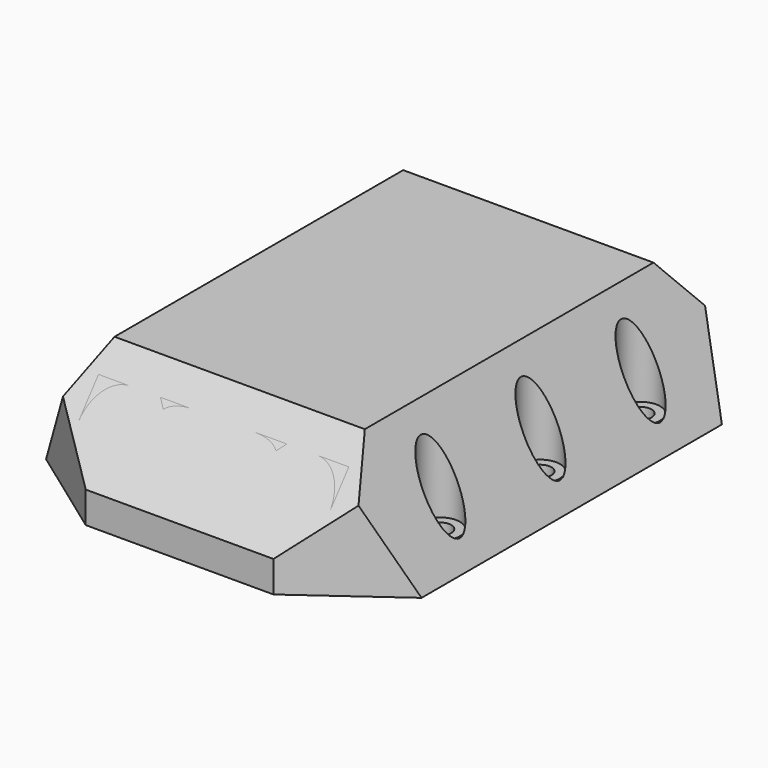
from build123d import *

# Parameters (mm, degrees)
F0_R         = 3.125
F1_DEPTH     = 20
F2_START     = 16
F2_DEPTH     = 4
F3_T1_DEPTH  = 163.5931549515
F4_SIZE2     = 15
F4_SIZE      = 12
F0_R_2       = 1.75
F5_DEPTH     = 4
F6_SIZE2     = 15
F6_SIZE      = 5
F7_T1_DEPTH  = 38.5354006484
F7_T6_DEPTH  = 25.1531696001
F7_T12_DEPTH = 74.7709385518
F7_T18_DEPTH = 25.1531696001
F7_T24_DEPTH = 25.1531696001
F7_T30_DEPTH = 74.7709385518
F7_T36_DEPTH = 25.1531696001


# Not quite as in the source:
# - a fillet or chamfer that OpenCascade refuses, or shapes differently, is made with other operations: its cross-section is extruded or revolved along the edge and cut away or added


with BuildPart() as f1:
    # F0 (on Top) → F1 (new body)
    with BuildSketch(Plane.XY):
        Polygon((-15, 40.8282039139), (-30, 30), (-30, -30), (-15, -40.8282039139), (15, -40.8282039139), (30, -30), (30, 30), (15, 40.8282039139), align=None)
        with Locations((-25, -20)):
            Circle(F0_R, mode=Mode.SUBTRACT)
        with Locations((25, -20)):
            Circle(F0_R, mode=Mode.SUBTRACT)
        with Locations((-25, 0)):
            Circle(F0_R, mode=Mode.SUBTRACT)
        with Locations((-25, 20)):
            Circle(F0_R, mode=Mode.SUBTRACT)
        Polygon((-11.7677003242, -30.8282039139), (-20, -24.8854692759), (-20, 24.8854692759), (-11.7677003242, 30.8282039139), (11.7677003242, 30.8282039139), (20, 24.8854692759), (20, -24.8854692759), (11.7677003242, -30.8282039139), align=None, mode=Mode.SUBTRACT)
        with Locations((25, 0)):
            Circle(F0_R, mode=Mode.SUBTRACT)
        with Locations((25, 20)):
            Circle(F0_R, mode=Mode.SUBTRACT)
    extrude(amount=F1_DEPTH)

    # F0 (on Top) → F2 (join)
    with BuildSketch(Plane.XY.offset(F2_START)):
        Polygon((-20, 24.8854692759), (-20, -24.8854692759), (-11.7677003242, -30.8282039139), (11.7677003242, -30.8282039139), (20, -24.8854692759), (20, 24.8854692759), (11.7677003242, 30.8282039139), (-11.7677003242, 30.8282039139), align=None)
    extrude(amount=F2_DEPTH)

    # F3: chamfer of 10 x 20 on 2 edges, made by hand

    # F3_s2 → F3_t1 (cut)
    with BuildSketch(Plane.XZ.offset(-81.7965774757)):
        Polygon((-30, 0), (-20, 20), (-30, 20), align=None)
        Polygon((20, 20), (30, 0), (30, 20), align=None)
    extrude(amount=F3_T1_DEPTH, mode=Mode.SUBTRACT)

    # F4
    f4_edges = [f1.edges().sort_by_distance(p)[0] for p in [
        (0, -40.828204, 20),
        (0, 40.828204, 20),
    ]]
    f4_side = f1.faces().sort_by_distance((0, 0, 20))[0]
    chamfer(f4_edges, length=F4_SIZE, length2=F4_SIZE2, reference=f4_side)

    # F0 (on Top) → F5 (join)
    with BuildSketch(Plane.XY):
        with Locations((25, -20)):
            Circle(F0_R)
        with Locations((25, -20)):
            Circle(F0_R_2, mode=Mode.SUBTRACT)
        with Locations((25, 0)):
            Circle(F0_R)
        with Locations((25, 0)):
            Circle(F0_R_2, mode=Mode.SUBTRACT)
        with Locations((25, 20)):
            Circle(F0_R)
        with Locations((25, 20)):
            Circle(F0_R_2, mode=Mode.SUBTRACT)
        with Locations((-25, -20)):
            Circle(F0_R)
        with Locations((-25, -20)):
            Circle(F0_R_2, mode=Mode.SUBTRACT)
        with Locations((-25, 0)):
            Circle(F0_R)
        with Locations((-25, 0)):
            Circle(F0_R_2, mode=Mode.SUBTRACT)
        with Locations((-25, 20)):
            Circle(F0_R)
        with Locations((-25, 20)):
            Circle(F0_R_2, mode=Mode.SUBTRACT)
    extrude(amount=F5_DEPTH)

    # F6
    f6_edges = [f1.edges().sort_by_distance(p)[0] for p in [
        (0, 30.828204, 0),
        (-15.88385, 27.856837, 0),
        (15.88385, 27.856837, 0),
        (0, -30.828204, 0),
        (-15.88385, -27.856837, 0),
        (15.88385, -27.856837, 0),
    ]]
    f6_side = f1.faces().sort_by_distance((-21.906907, 34.592507, 0))[0]
    chamfer(f6_edges, length=F6_SIZE, length2=F6_SIZE2, reference=f6_side)

    # F7: fillet of radius 5 on 8 edges, made by hand

    # F7_s2 → F7_t1 (join)
    with BuildSketch(Plane.YZ.offset(-19.2677003242)):
        with BuildLine():
            ThreePointArc((-27.8282039139, 16), (-29.4093427439, 15.7434164903), (-30.8282039139, 15))
            Line((-30.8282039139, 15), (-30.8282039139, 16))
            Line((-30.8282039139, 16), (-27.8282039139, 16))
        make_face()
        with BuildLine():
            ThreePointArc((27.8282039139, 16), (29.4093427439, 15.7434164903), (30.8282039139, 15))
            Line((30.8282039139, 15), (30.8282039139, 16))
            Line((30.8282039139, 16), (27.8282039139, 16))
        make_face()
    extrude(amount=F7_T1_DEPTH)


with BuildPart() as f7_tool4:
    # F7_s5 → F7_t6 (new body)
    with BuildSketch(Plane(origin=(12.9751018297, 9.3664698943, 0), x_dir=(0, 0, 1), z_dir=(-0.8108108108, -0.5853083197, 0))):
        with BuildLine():
            ThreePointArc((15, 31.8835739144), (15.7434164903, 30.4647127444), (16, 28.8835739144))
            Line((16, 28.8835739144), (16, 31.8835739144))
            Line((16, 31.8835739144), (15, 31.8835739144))
        make_face()
    extrude(amount=F7_T6_DEPTH)

    split(bisect_by=Plane.YZ.offset(-20), keep=Keep.TOP)

    split(bisect_by=Plane(origin=(0, 27.3342706792, 21.8674165433), x_dir=(1, 0, 0), z_dir=(0, -0.7808688094, -0.6246950476)), keep=Keep.TOP)


with BuildPart() as f1_1:
    add(f1.part)

    # F7_t3: union F7_tool4
    add(f7_tool4.part)


with BuildPart() as f7_tool10:
    # F7_s11 → F7_t12 (new body)
    with BuildSketch(Plane.XZ.offset(-37.3854692759)):
        with BuildLine():
            ThreePointArc((-20, 11), (-18.5355339059, 14.5355339059), (-15, 16))
            Line((-15, 16), (-20, 16))
            Line((-20, 16), (-20, 11))
        make_face()
    extrude(amount=F7_T12_DEPTH)

    split(bisect_by=Plane(origin=(0, 27.3342706792, 21.8674165433), x_dir=(1, 0, 0), z_dir=(0, -0.7808688094, -0.6246950476)), keep=Keep.TOP)

    split(bisect_by=Plane(origin=(0, -27.3342706792, 21.8674165433), x_dir=(1, 0, 0), z_dir=(0, 0.7808688094, -0.6246950476)), keep=Keep.TOP)


with BuildPart() as f1_2:
    add(f1_1.part)

    # F7_t9: union F7_tool10
    add(f7_tool10.part)


with BuildPart() as f7_tool16:
    # F7_s17 → F7_t18 (new body)
    with BuildSketch(Plane(origin=(-7.4193600083, 5.3558895387, 0), x_dir=(0, 0, 1), z_dir=(0.8108108108, -0.5853083197, 0))):
        with BuildLine():
            ThreePointArc((16, 28.8835739144), (15.7434164903, 30.4647127444), (15, 31.8835739144))
            Line((15, 31.8835739144), (16, 31.8835739144))
            Line((16, 31.8835739144), (16, 28.8835739144))
        make_face()
    extrude(amount=F7_T18_DEPTH)

    split(bisect_by=Plane.YZ.offset(-20), keep=Keep.TOP)

    split(bisect_by=Plane(origin=(0, -27.3342706792, 21.8674165433), x_dir=(1, 0, 0), z_dir=(0, 0.7808688094, -0.6246950476)), keep=Keep.TOP)


with BuildPart() as f1_3:
    add(f1_2.part)

    # F7_t15: union F7_tool16
    add(f7_tool16.part)


with BuildPart() as f7_tool22:
    # F7_s23 → F7_t24 (new body)
    with BuildSketch(Plane(origin=(-12.9751018297, -9.3664698943, 0), x_dir=(0, 0, 1), z_dir=(0.8108108108, 0.5853083197, 0))):
        with BuildLine():
            ThreePointArc((16, 28.8835739144), (15.7434164903, 30.4647127444), (15, 31.8835739144))
            Line((15, 31.8835739144), (16, 31.8835739144))
            Line((16, 31.8835739144), (16, 28.8835739144))
        make_face()
    extrude(amount=F7_T24_DEPTH)

    split(bisect_by=Plane.YZ.offset(20), keep=Keep.BOTTOM)

    split(bisect_by=Plane(origin=(0, -27.3342706792, 21.8674165433), x_dir=(1, 0, 0), z_dir=(0, 0.7808688094, -0.6246950476)), keep=Keep.TOP)


with BuildPart() as f1_4:
    add(f1_3.part)

    # F7_t21: union F7_tool22
    add(f7_tool22.part)


with BuildPart() as f7_tool28:
    # F7_s29 → F7_t30 (new body)
    with BuildSketch(Plane.XZ.offset(37.3854692759)):
        with BuildLine():
            ThreePointArc((20, 11), (18.5355339059, 14.5355339059), (15, 16))
            Line((15, 16), (20, 16))
            Line((20, 16), (20, 11))
        make_face()
    extrude(amount=-F7_T30_DEPTH)

    split(bisect_by=Plane(origin=(0, 27.3342706792, 21.8674165433), x_dir=(1, 0, 0), z_dir=(0, -0.7808688094, -0.6246950476)), keep=Keep.TOP)

    split(bisect_by=Plane(origin=(0, -27.3342706792, 21.8674165433), x_dir=(1, 0, 0), z_dir=(0, 0.7808688094, -0.6246950476)), keep=Keep.TOP)


with BuildPart() as f1_5:
    add(f1_4.part)

    # F7_t27: union F7_tool28
    add(f7_tool28.part)


with BuildPart() as f7_tool34:
    # F7_s35 → F7_t36 (new body)
    with BuildSketch(Plane(origin=(7.4193600083, -5.3558895387, 0), x_dir=(0, 0, 1), z_dir=(-0.8108108108, 0.5853083197, 0))):
        with BuildLine():
            ThreePointArc((16, 28.8835739144), (15.7434164903, 30.4647127444), (15, 31.8835739144))
            Line((15, 31.8835739144), (16, 31.8835739144))
            Line((16, 31.8835739144), (16, 28.8835739144))
        make_face()
    extrude(amount=F7_T36_DEPTH)

    split(bisect_by=Plane.YZ.offset(20), keep=Keep.BOTTOM)

    split(bisect_by=Plane(origin=(0, 27.3342706792, 21.8674165433), x_dir=(1, 0, 0), z_dir=(0, -0.7808688094, -0.6246950476)), keep=Keep.TOP)


with BuildPart() as f1_6:
    add(f1_5.part)

    # F7_t33: union F7_tool34
    add(f7_tool34.part)


solid = f1_6.part
